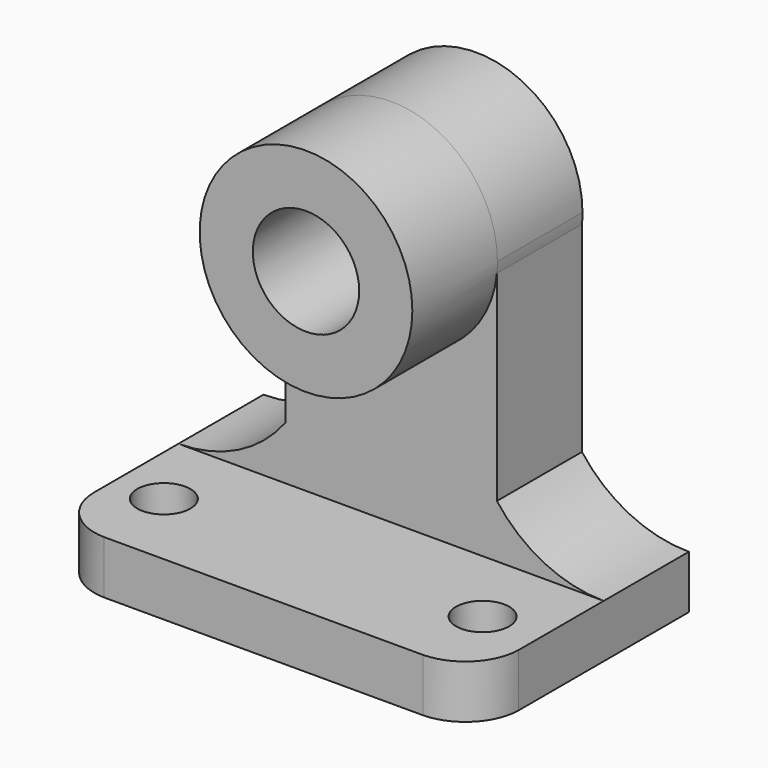
from build123d import *
from build123d import SkipClean  # not in build123d's __all__

# Parameters (mm, degrees)
F0_W      = 50.8
F0_H      = 31.75
F1_DEPTH  = 6.35
F2_W      = 50.8
F2_H      = 12.7
F3_DEPTH  = 44.45
F4_R      = 12.7
F5_DEPTH  = 12.7
F6_R      = 6.35
F7_DEPTH  = 12.7
F8_R      = 3.175
F9_DEPTH  = 25.4
F11_DEPTH = 25.4
F13_DEPTH = 25.4


with BuildPart() as f1:
    # F0 (on Top) → F1 (new body)
    with BuildSketch(Plane.XY):
        with Locations((25.4, 15.875)):
            Rectangle(F0_W, F0_H)
    extrude(amount=F1_DEPTH)

    # F2 (on face) → F3 (join)
    with BuildSketch(Plane.XY.offset(6.35)):
        with Locations((25.4, 25.4)):
            Rectangle(F2_W, F2_H)
    extrude(amount=F3_DEPTH)

    # F4 (on face) → F5 (join)
    with BuildSketch(Plane.XZ.offset(-19.05)):
        with Locations((25.4, 37.9059378386)):
            Circle(F4_R)
    extrude(amount=F5_DEPTH)

    # F6 (on face) → F7 (cut)
    with BuildSketch(Plane.XZ.offset(-6.35)):
        with Locations((25.4, 37.9059378386)):
            Circle(F6_R)
    extrude(amount=-F7_DEPTH, mode=Mode.SUBTRACT)

    # F8 (on face) → F9 (cut)
    with BuildSketch(Plane.XY.offset(6.35)):
        with Locations((5.8808145113, 9.525)):
            Circle(F8_R)
        with Locations((43.9513325691, 9.525)):
            Circle(F8_R)
    extrude(amount=-F9_DEPTH, mode=Mode.SUBTRACT)

    # F10 (on face) → F11 (cut)
    with BuildSketch(Plane.XY.offset(6.35)):
        with BuildLine():
            ThreePointArc((50.8, 6.35), (48.9094635793, 1.8905364207), (44.45, 0))
            Line((44.45, 0), (50.8, 0))
            Line((50.8, 0), (50.8, 6.35))
        make_face()
        with BuildLine():
            ThreePointArc((6.35, 0), (1.9050641376, 1.9050641376), (0, 6.35))
            Line((0, 6.35), (0, 0))
            Line((0, 0), (6.35, 0))
        make_face()
    extrude(amount=-F11_DEPTH, mode=Mode.SUBTRACT)

    # F12 (on face) → F13 (cut)
    with BuildSketch(Plane.XZ.offset(-19.05)):
        with BuildLine():
            ThreePointArc((38.1, 37.9059378386), (38.084216594, 37.2729691208), (38.0369056067, 36.6415736948))
            Line((38.0369056067, 36.6415736948), (38.0369056067, 12.7))
            ThreePointArc((38.0369056067, 12.7), (43.6722535382, 8.0251871407), (50.8, 6.35))
            Line((50.8, 6.35), (50.8, 50.8))
            Line((50.8, 50.8), (0, 50.8))
            Line((0, 50.8), (0, 6.35))
            ThreePointArc((0, 6.35), (7.1277464618, 8.0251871407), (12.7630943933, 12.7))
            Line((12.7630943933, 12.7), (12.7630943933, 36.6415736948))
            ThreePointArc((12.7630943933, 36.6415736948), (24.7670312823, 50.5901544325), (38.1, 37.9059378386))
        make_face()
    with SkipClean():  # cleaning this boolean's faces spoils the solid; the shape is the same uncleaned
        extrude(amount=-F13_DEPTH, mode=Mode.SUBTRACT)


solid = f1.part
